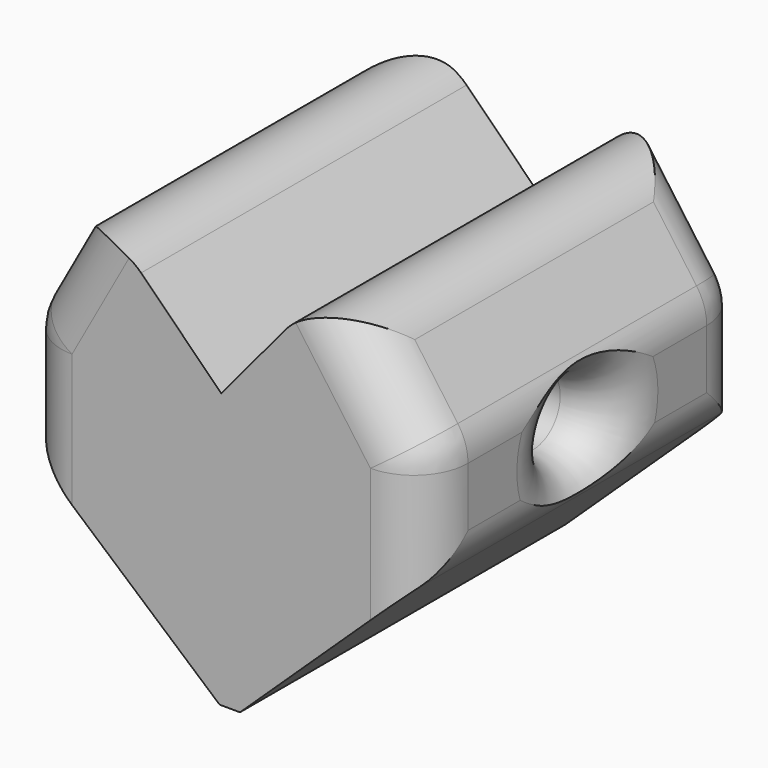
from build123d import *

# Parameters (mm, degrees)
F1_DEPTH     = 38.1
F3_DEPTH     = 38.1
F5_D         = 6.35
F6_T1_DEPTH  = 20.7437886812
F6_T3_DEPTH  = 27.94
F6_T5_DEPTH  = 49.7055689591
F6_T7_DEPTH  = 20.4179452734
F6_T9_DEPTH  = 49.0300859467
F6_T11_DEPTH = 71.8058781858
F6_T13_DEPTH = 25.3882661408
F6_T15_DEPTH = 70.8375780274
F6_T17_DEPTH = 26.1528668654
F6_T22_DEPTH = 5.08
F6_T28_DEPTH = 5.08
F6_T34_DEPTH = 5.08
F6_T40_DEPTH = 5.08


# Not quite as in the source:
# - a fillet or chamfer that OpenCascade refuses, or shapes differently, is made with other operations: its cross-section is extruded or revolved along the edge and cut away or added


with BuildPart() as f1:
    # F0 (on Front) → F1 (new body)
    with BuildSketch(Plane.XZ):
        Polygon((0, 38.1), (0, 0.2683098665), (38.1, 0), (38.1, 38.1), align=None)
    extrude(amount=F1_DEPTH)

    # F2 (on face) → F3 (cut)
    with BuildSketch(Plane.XZ.offset(38.1)):
        Polygon((29.289287496, 38.1), (6.7755630988, 38.1), (19.05, 25.849385187), align=None)
        Polygon((0, 38.1), (0, 25.849385187), (6.7755630988, 38.1), align=None)
        Polygon((29.289287496, 38.1), (38.1, 25.849385187), (38.1, 38.1), align=None)
        Polygon((0, 0.2683098665), (18.8937886297, 0.1352550134), (0, 16.4943691343), align=None)
        Polygon((38.1, 16.4943691343), (20.8069253196, 0.1217822194), (38.1, 0), align=None)
    extrude(amount=-F3_DEPTH, mode=Mode.SUBTRACT)

    # F5 (through all)
    with Locations(Plane.YZ.offset(38.1)):
        with Locations((-19.05, 21.1718771607)):
            Hole(F5_D / 2)

    # F6: fillet of radius 5.08 on 16 edges, made by hand

    # F6_s2 → F6_t1 (cut)
    with BuildSketch(Plane.XY.offset(3.7943691343)):
        with BuildLine():
            ThreePointArc((5.08, 0), (1.4878975516, -1.4878975516), (0, -5.08))
            Line((0, -5.08), (0, 0))
            Line((0, 0), (5.08, 0))
        make_face()
        with BuildLine():
            ThreePointArc((5.08, -38.1), (1.4878975516, -36.6121024484), (0, -33.02))
            Line((0, -33.02), (0, -38.1))
            Line((0, -38.1), (5.08, -38.1))
        make_face()
    extrude(amount=F6_T1_DEPTH, mode=Mode.SUBTRACT)

    # F6_s4 → F6_t3 (cut)
    with BuildSketch(Plane.XZ.offset(5.08)):
        with BuildLine():
            ThreePointArc((0.634616087, 26.9968082311), (0.1612120254, 25.8077738444), (0, 24.5381578155))
            Line((0, 24.5381578155), (0, 25.849385187))
            Line((0, 25.849385187), (0.634616087, 26.9968082311))
        make_face()
        with BuildLine():
            ThreePointArc((37.1441471446, 27.1784247107), (37.8551353391, 25.7704755844), (38.1, 24.2123144077))
            Line((38.1, 24.2123144077), (38.1, 25.849385187))
            Line((38.1, 25.849385187), (37.1441471446, 27.1784247107))
        make_face()
    extrude(amount=F6_T3_DEPTH, mode=Mode.SUBTRACT)

    # F6_s6 → F6_t5 (cut)
    with BuildSketch(Plane.XZ.offset(-5.8027844796)):
        with BuildLine():
            ThreePointArc((1.754752754, 14.9750232202), (0.4594666969, 16.704305057), (0, 18.8154829261))
            Line((0, 18.8154829261), (0, 16.4943691343))
            Line((0, 16.4943691343), (1.754752754, 14.9750232202))
        make_face()
    extrude(amount=F6_T5_DEPTH, mode=Mode.SUBTRACT)

    # F6_s8 → F6_t7 (cut)
    with BuildSketch(Plane.XY.offset(3.7943691343)):
        with BuildLine():
            ThreePointArc((33.02, 0), (36.6121024484, -1.4878975516), (38.1, -5.08))
            Line((38.1, -5.08), (38.1, 0))
            Line((38.1, 0), (33.02, 0))
        make_face()
        with BuildLine():
            ThreePointArc((33.02, -38.1), (36.6121024484, -36.6121024484), (38.1, -33.02))
            Line((38.1, -33.02), (38.1, -38.1))
            Line((38.1, -38.1), (33.02, -38.1))
        make_face()
    extrude(amount=F6_T7_DEPTH, mode=Mode.SUBTRACT)

    # F6_s10 → F6_t9 (cut)
    with BuildSketch(Plane.XZ.offset(-5.4650429733)):
        with BuildLine():
            ThreePointArc((38.1, 18.6803863236), (37.6863002203, 16.6723917386), (36.5125817899, 14.991447121))
            Line((36.5125817899, 14.991447121), (38.1, 16.4943691343))
            Line((38.1, 16.4943691343), (38.1, 18.6803863236))
        make_face()
    extrude(amount=F6_T9_DEPTH, mode=Mode.SUBTRACT)

    # F6_s12 → F6_t11 (cut)
    with BuildSketch(Plane.XZ.offset(-16.8529390929)):
        with BuildLine():
            ThreePointArc((11.5469219559, 33.3379013421), (7.2465010014, 34.7721948924), (3.5129264291, 32.2009618637))
            Line((3.5129264291, 32.2009618637), (6.7755630988, 38.1))
            Line((6.7755630988, 38.1), (11.5469219559, 33.3379013421))
        make_face()
    extrude(amount=F6_T11_DEPTH, mode=Mode.SUBTRACT)

    # F6_s14 → F6_t13 (cut)
    with BuildSketch(Plane(origin=(11.5824663758, 0, 20.9417773971), x_dir=(0, 1, 0), z_dir=(0.4839863023, 0, 0.8750755734))):
        with BuildLine():
            ThreePointArc((-38.1, 7.4307483528), (-36.6121024484, 11.0228508012), (-33.02, 12.5107483528))
            Line((-33.02, 12.5107483528), (-38.1, 12.5107483528))
            Line((-38.1, 12.5107483528), (-38.1, 7.4307483528))
        make_face()
        with BuildLine():
            ThreePointArc((0, 7.4307483528), (-1.4878975516, 11.0228508012), (-5.08, 12.5107483528))
            Line((-5.08, 12.5107483528), (0, 12.5107483528))
            Line((0, 12.5107483528), (0, 7.4307483528))
        make_face()
    extrude(amount=F6_T13_DEPTH, mode=Mode.SUBTRACT)

    # F6_s16 → F6_t15 (cut)
    with BuildSketch(Plane.XZ.offset(-16.3687890137)):
        with BuildLine():
            ThreePointArc((25.0903071925, 33.076204123), (29.1727291737, 34.8949986115), (33.1122507828, 32.7844650022))
            Line((33.1122507828, 32.7844650022), (29.289287496, 38.1))
            Line((29.289287496, 38.1), (25.0903071925, 33.076204123))
        make_face()
    extrude(amount=F6_T15_DEPTH, mode=Mode.SUBTRACT)

    # F6_s18 → F6_t17 (cut)
    with BuildSketch(Plane(origin=(-15.4901461094, 0, 21.5378510306), x_dir=(0, 1, 0), z_dir=(0.5838799809, 0, -0.8118399891))):
        with BuildLine():
            ThreePointArc((-33.02, 46.024042114), (-36.6121024484, 44.5361445625), (-38.1, 40.944042114))
            Line((-38.1, 40.944042114), (-38.1, 46.024042114))
            Line((-38.1, 46.024042114), (-33.02, 46.024042114))
        make_face()
        with BuildLine():
            ThreePointArc((-5.08, 46.024042114), (-1.4878975516, 44.5361445625), (0, 40.944042114))
            Line((0, 40.944042114), (0, 46.024042114))
            Line((0, 46.024042114), (-5.08, 46.024042114))
        make_face()
    extrude(amount=F6_T17_DEPTH, mode=Mode.SUBTRACT)


with BuildPart() as f6_tool20:
    # F6_s21 → F6_t22 (new body)
    with BuildSketch(Plane.XZ.offset(5.08)):
        Polygon((5.08, 24.5381578155), (0.634616087, 26.9968082311), (0, 25.849385187), (0, 24.5381578155), align=None)
    extrude(amount=-F6_T22_DEPTH)

    # F6_s23 → F6_t24 (revolve, cut)
    with BuildSketch(Plane(origin=(5.08, -5.08, 24.5381578155), x_dir=(0.9682653493, 0, -0.2499244151), z_dir=(0.2499244151, 0, 0.9682653493))):
        with BuildLine():
            ThreePointArc((0, -5.08), (5.08, 0), (0, 5.08))
            Line((0, 5.08), (0, -5.08))
        make_face()
    revolve(axis=Axis((5.08, -5.08, 24.5381578155), (0, 1, 0)), mode=Mode.SUBTRACT)


with BuildPart() as f1_1:
    add(f1.part)

    # F6_t19: cut F6_tool20
    add(f6_tool20.part, mode=Mode.SUBTRACT)


with BuildPart() as f6_tool26:
    # F6_s27 → F6_t28 (new body)
    with BuildSketch(Plane.XZ.offset(33.02)):
        Polygon((5.08, 24.5381578155), (0.634616087, 26.9968082311), (0, 25.849385187), (0, 24.5381578155), align=None)
    extrude(amount=F6_T28_DEPTH)

    # F6_s29 → F6_t30 (revolve, cut)
    with BuildSketch(Plane(origin=(5.08, -33.02, 24.5381578155), x_dir=(0.9682653493, 0, -0.2499244151), z_dir=(-0.2499244151, 0, -0.9682653493))):
        with BuildLine():
            ThreePointArc((0, -5.08), (5.08, 0), (0, 5.08))
            Line((0, 5.08), (0, -5.08))
        make_face()
    revolve(axis=Axis((5.08, -33.02, 24.5381578155), (0, -1, 0)), mode=Mode.SUBTRACT)


with BuildPart() as f1_2:
    add(f1_1.part)

    # F6_t25: cut F6_tool26
    add(f6_tool26.part, mode=Mode.SUBTRACT)


with BuildPart() as f6_tool32:
    # F6_s33 → F6_t34 (new body)
    with BuildSketch(Plane.XZ.offset(5.08)):
        Polygon((33.02, 24.2123144077), (38.1, 24.2123144077), (38.1, 25.849385187), (37.1441471446, 27.1784247107), align=None)
    extrude(amount=-F6_T34_DEPTH)

    # F6_s35 → F6_t36 (revolve, cut)
    with BuildSketch(Plane(origin=(33.02, -5.08, 24.2123144077), x_dir=(-0.9517982951, 0, -0.3067246411), z_dir=(0.3067246411, 0, -0.9517982951))):
        with BuildLine():
            ThreePointArc((0, -5.08), (5.08, 0), (0, 5.08))
            Line((0, 5.08), (0, -5.08))
        make_face()
    revolve(axis=Axis((33.02, -5.08, 24.2123144077), (0, 1, 0)), mode=Mode.SUBTRACT)


with BuildPart() as f1_3:
    add(f1_2.part)

    # F6_t31: cut F6_tool32
    add(f6_tool32.part, mode=Mode.SUBTRACT)


with BuildPart() as f6_tool38:
    # F6_s39 → F6_t40 (new body)
    with BuildSketch(Plane.XZ.offset(33.02)):
        Polygon((33.02, 24.2123144077), (38.1, 24.2123144077), (38.1, 25.849385187), (37.1441471446, 27.1784247107), align=None)
    extrude(amount=F6_T40_DEPTH)

    # F6_s41 → F6_t42 (revolve, cut)
    with BuildSketch(Plane(origin=(33.02, -33.02, 24.2123144077), x_dir=(-0.9517982951, 0, -0.3067246411), z_dir=(-0.3067246411, 0, 0.9517982951))):
        with BuildLine():
            ThreePointArc((0, -5.08), (5.08, 0), (0, 5.08))
            Line((0, 5.08), (0, -5.08))
        make_face()
    revolve(axis=Axis((33.02, -33.02, 24.2123144077), (0, -1, 0)), mode=Mode.SUBTRACT)


with BuildPart() as f1_4:
    add(f1_3.part)

    # F6_t37: cut F6_tool38
    add(f6_tool38.part, mode=Mode.SUBTRACT)

    # F6_s43 → F6_t44 (revolve, cut)
    with BuildSketch(Plane.XY.offset(21.1718771607)):
        with BuildLine():
            ThreePointArc((0, -10.795), (1.4878975516, -14.3871024484), (5.08, -15.875))
            Line((5.08, -15.875), (0, -15.875))
            Line((0, -15.875), (0, -10.795))
        make_face()
    revolve(axis=Axis((0, -19.05, 21.1718771607), (1, 0, 0)), mode=Mode.SUBTRACT)

    # F6_s45 → F6_t46 (revolve, cut)
    with BuildSketch(Plane.XY.offset(21.1718771607)):
        with BuildLine():
            ThreePointArc((38.1, -10.795), (36.6121024484, -14.3871024484), (33.02, -15.875))
            Line((33.02, -15.875), (38.1, -15.875))
            Line((38.1, -15.875), (38.1, -10.795))
        make_face()
    revolve(axis=Axis((38.1, -19.05, 21.1718771607), (1, 0, 0)), mode=Mode.SUBTRACT)


solid = f1_4.part
